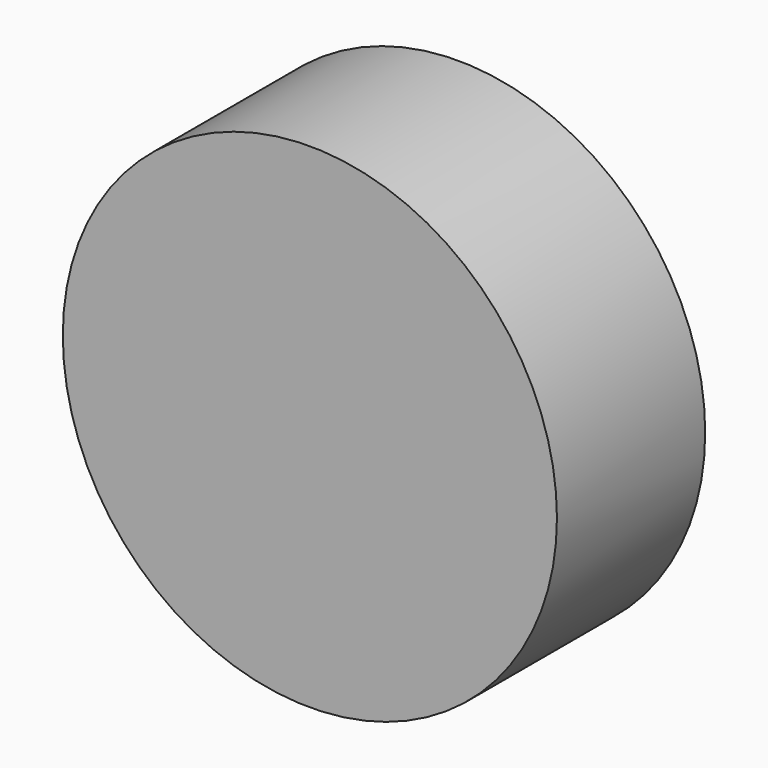
from build123d import *

# Parameters (mm, degrees)
F0_R     = 12.7
F1_DEPTH = 9.525


# Not quite as in the source:
# - a length typed as a fraction of an inch, garbled in the dataset ("3 / 203.2 mm" for 3/8 in), is restored


with BuildPart() as f1:
    # F0 (on Front) → F1 (new body)
    with BuildSketch(Plane.XZ):
        Circle(F0_R)
    extrude(amount=F1_DEPTH)


solid = f1.part
